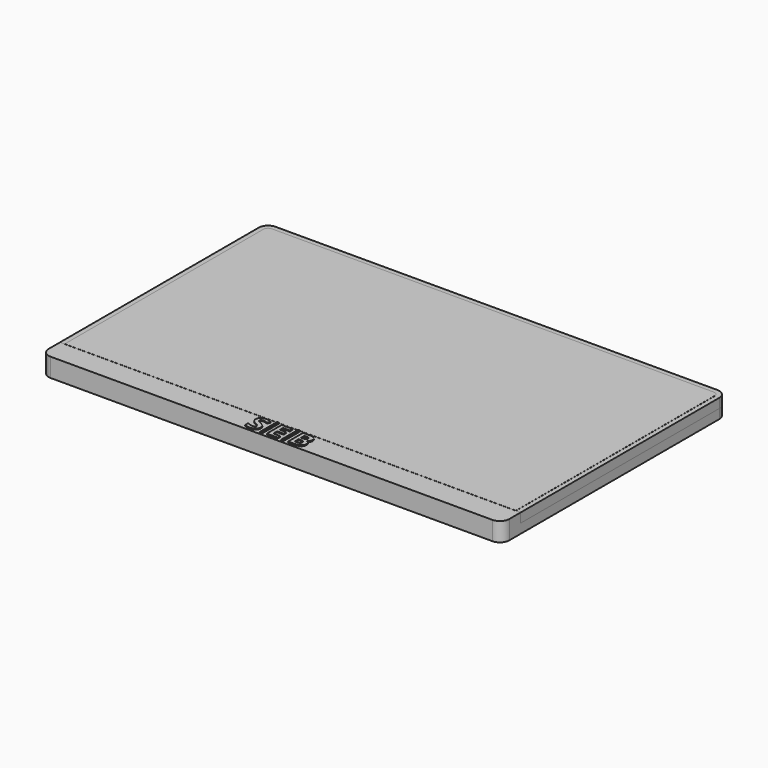
from build123d import *

# Parameters (mm, degrees)
F1_DEPTH     = 20
F3_DEPTH     = 10
F5_DEPTH     = 10
F7_DEPTH     = 0.1
F8_W         = 2
F8_H         = 23.2552895225
F8_TEXT_SIZE = 27.7777777778
F9_DEPTH     = 1


# Not quite as in the source:
# - Text() gives the source's letters only with a copy of the font that has no kerning and outlines rounded to 1/6400 em; it was checked with that copy


with BuildPart() as f1:
    # F0 (on Top) → F1 (new body)
    with BuildSketch(Plane.XY):
        with BuildLine():
            Line((235.15, 149.7), (-235.15, 149.7))
            ThreePointArc((-235.15, 149.7), (-242.2210678119, 146.7710678119), (-245.15, 139.7))
            Line((-245.15, 139.7), (-245.15, -139.7))
            ThreePointArc((-245.15, -139.7), (-242.2210678119, -146.7710678119), (-235.15, -149.7))
            Line((-235.15, -149.7), (235.15, -149.7))
            ThreePointArc((235.15, -149.7), (242.2210678119, -146.7710678119), (245.15, -139.7))
            Line((245.15, -139.7), (245.15, 139.7))
            ThreePointArc((245.15, 139.7), (242.2210678119, 146.7710678119), (235.15, 149.7))
        make_face()
    extrude(amount=F1_DEPTH)

    # F2 (on face) → F3 (cut)
    with BuildSketch(Plane.XY.offset(20)):
        with BuildLine():
            Line((-245.15, 139.7), (-245.15, -124.7))
            Line((-245.15, -124.7), (245.15, -124.7))
            Line((245.15, -124.7), (245.15, 139.7))
            ThreePointArc((245.15, 139.7), (242.2210678119, 146.7710678119), (235.15, 149.7))
            Line((235.15, 149.7), (-235.15, 149.7))
            ThreePointArc((-235.15, 149.7), (-242.2210678119, 146.7710678119), (-245.15, 139.7))
        make_face()
    extrude(amount=-F3_DEPTH, mode=Mode.SUBTRACT)


with BuildPart() as f5:
    # F4 (on face) → F5 (new body)
    with BuildSketch(Plane.XY.offset(10)):
        with BuildLine():
            Line((-245.15, -124.7), (245.15, -124.7))
            Line((245.15, -124.7), (245.15, 139.7))
            ThreePointArc((245.15, 139.7), (242.2210678119, 146.7710678119), (235.15, 149.7))
            Line((235.15, 149.7), (-235.15, 149.7))
            ThreePointArc((-235.15, 149.7), (-242.2210678119, 146.7710678119), (-245.15, 139.7))
            Line((-245.15, 139.7), (-245.15, -124.7))
        make_face()
    extrude(amount=F5_DEPTH)


with BuildPart() as f7:
    # F6 (on face) → F7 (new body)
    with BuildSketch(Plane.XY.offset(20)):
        with BuildLine():
            Line((-240.15, -124.7), (240.15, -124.7))
            Line((240.15, -124.7), (240.15, 139.7))
            ThreePointArc((240.15, 139.7), (238.6855339059, 143.2355339059), (235.15, 144.7))
            Line((235.15, 144.7), (-235.15, 144.7))
            ThreePointArc((-235.15, 144.7), (-238.6855339059, 143.2355339059), (-240.15, 139.7))
            Line((-240.15, 139.7), (-240.15, -124.7))
        make_face()
    extrude(amount=F7_DEPTH)


with BuildPart() as f9:
    # F8 (on face) → F9 (new body)
    with BuildSketch(Plane.XY.offset(20)):
        with Locations((-12.5, -137)):
            Rectangle(F8_W, F8_H)
        with Locations((10, -137)):
            Rectangle(F8_W, F8_H)
        with Locations((-32.1462673611, -147)):
            Text('S E B', F8_TEXT_SIZE, font='Open Sans', font_style=FontStyle.BOLD, text_align=(TextAlign.LEFT, TextAlign.BOTTOM))
    extrude(amount=F9_DEPTH)


solid = Compound([f1.part, f5.part, f7.part, f9.part])
